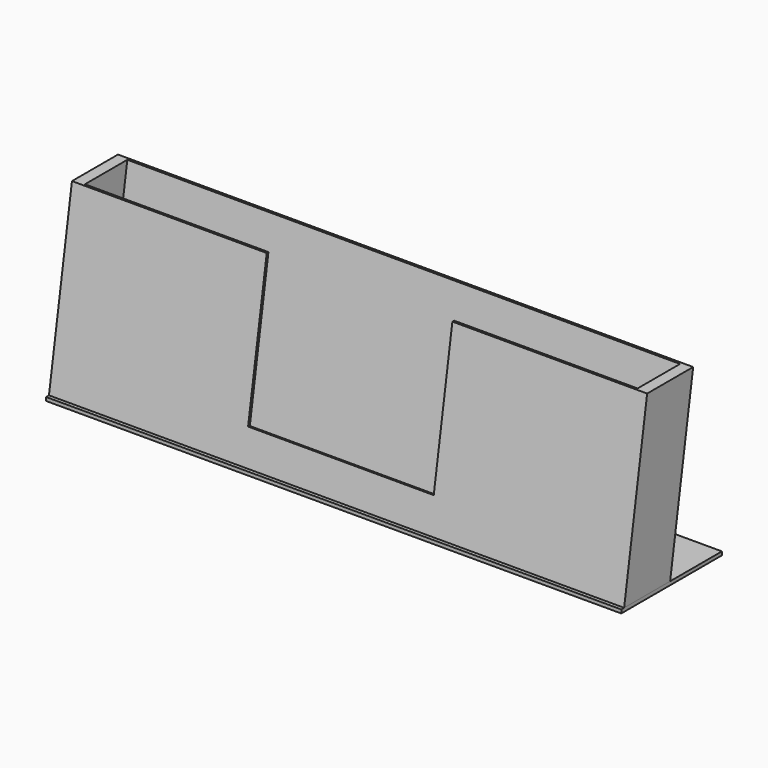
from build123d import *
from build123d import SkipClean  # not in build123d's __all__

# Parameters (mm, degrees)
F1_W      = 81.28
F1_H      = 8.128
F2_W      = 81.28
F2_H      = 8.128
F4_W      = 26.233073324
F4_H      = 20.56436991
F5_DEPTH  = 1
F6_W      = 78.105
F6_H      = 7.493
F7_W      = 78.105
F7_H      = 7.493
F9_W      = 81.28
F9_H      = 17.78
F10_DEPTH = 0.5


with BuildPart() as f3:
    # F1 (on Top) → F3 section 0
    with BuildSketch(Plane.XY):
        Rectangle(F1_W, F1_H)
    # F2 (on offset) → F3 section 1
    with BuildSketch(Plane.XY.offset(25)):
        with Locations((0, 4.064)):
            Rectangle(F2_W, F2_H)
    loft()

    # F4 (on face) → F5 (cut)
    with BuildSketch(Plane(origin=(0, -3.9593706469, 0.6436352924), x_dir=(1, 0, 0), z_dir=(0, -0.9870433569, 0.1604537681))):
        with Locations((0, 14.4417314122)):
            Rectangle(F4_W, F4_H)
    extrude(amount=-F5_DEPTH, mode=Mode.SUBTRACT)

    # F6 (on offset) → F8 section 0
    with BuildSketch(Plane.XY.offset(25)):
        with Locations((-1.3208e-06, 4.0446073394)):
            Rectangle(F6_W, F6_H)
    # F7 (on Top) → F8 section 1
    with BuildSketch(Plane.XY):
        Rectangle(F7_W, F7_H)
    loft(mode=Mode.SUBTRACT)

    # F9 (on Top) → F10 (join)
    with BuildSketch(Plane.XY):
        with Locations((-2.539e-07, 4.3180031988)):
            Rectangle(F9_W, F9_H)
    with SkipClean():  # cleaning this boolean's faces spoils the solid; the shape is the same uncleaned
        extrude(amount=-F10_DEPTH)


solid = f3.part
